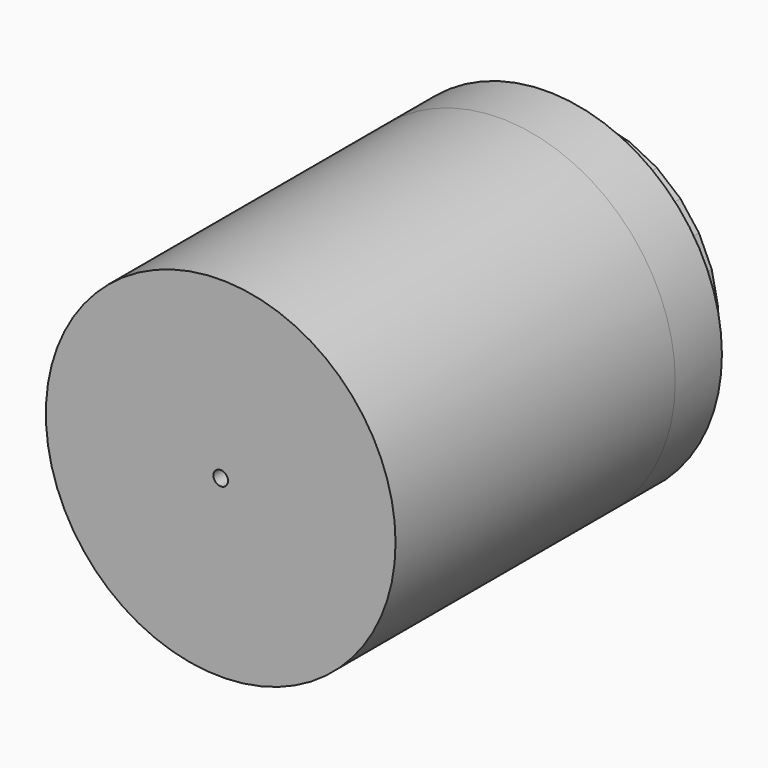
from build123d import *

# Parameters (mm, degrees)
F0_R     = 76.2
F2_DEPTH = 177.8
F1_R     = 76.2
F3_DEPTH = 25.4
F5_DEPTH = 19.05
F9_D     = 6.35
F9_2_D   = 6.35
F9_3_D   = 6.35


# Not quite as in the source:
# - the program builds the solid bodies; features that only make, move or delete a surface that nothing else refers to are left out


with BuildPart() as f2:
    # F0 (on Front) → F2 (new body)
    with BuildSketch(Plane.XZ):
        Circle(F0_R)
    extrude(amount=F2_DEPTH)

    # F9 (through all)
    with Locations(Plane(origin=(0, 19.05, 0), x_dir=(-1, 0, 0), z_dir=(0, 1, 0))):
        with Locations((0, 0)):
            Hole(F9_D / 2)


with BuildPart() as f3:
    # F1 (on face) → F3 (new body)
    with BuildSketch(Plane.XZ):
        Circle(F1_R)
    extrude(amount=F3_DEPTH)

    # F9#2 (through all)
    with Locations(Plane(origin=(0, 19.05, 0), x_dir=(-1, 0, 0), z_dir=(0, 1, 0))):
        with Locations((0, 0)):
            Hole(F9_2_D / 2)


with BuildPart() as f5:
    # F4 (on face) → F5 (new body)
    with BuildSketch(Plane(origin=(0, 0, 0), x_dir=(-1, 0, 0), z_dir=(0, 1, 0))):
        Polygon((49.6898963324, 32.6336398575), (41.1823988684, 42.8724885133), (30.6098439624, 50.961531575), (18.5023836646, 56.4951506468), (5.4671365906, 59.1958669619), (-7.8422555409, 58.9282553272), (-20.7584042331, 55.7057349074), (-32.6336398575, 49.6898963324), (-42.8724885133, 41.1823988684), (-50.961531575, 30.6098439624), (-56.4951506468, 18.5023836646), (-59.1958669619, 5.4671365906), (-58.9282553272, -7.8422555409), (-55.7057349074, -20.7584042331), (-49.6898963324, -32.6336398575), (-41.1823988684, -42.8724885133), (-30.6098439624, -50.961531575), (-18.5023836646, -56.4951506468), (-5.4671365906, -59.1958669619), (7.8422555409, -58.9282553272), (20.7584042331, -55.7057349074), (32.6336398575, -49.6898963324), (42.8724885133, -41.1823988684), (50.961531575, -30.6098439624), (56.4951506468, -18.5023836646), (59.1958669619, -5.4671365906), (58.9282553272, 7.8422555409), (55.7057349074, 20.7584042331), align=None)
    extrude(amount=F5_DEPTH)

    # F9#3 (through all)
    with Locations(Plane(origin=(0, 19.05, 0), x_dir=(-1, 0, 0), z_dir=(0, 1, 0))):
        with Locations((0, 0)):
            Hole(F9_3_D / 2)


solid = Compound([f2.part, f3.part, f5.part])
